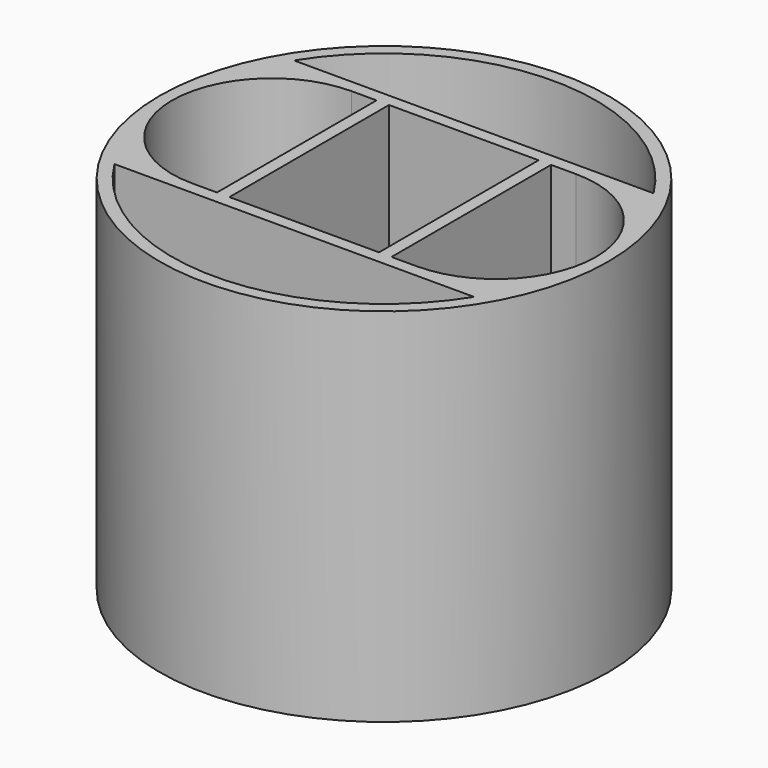
from build123d import *

# Parameters (mm, degrees)
F2_R     = 57.15
F3_DEPTH = 88.9
F0_R     = 57.15
F1_DEPTH = 3.175


# Not quite as in the source:
# - a feature names something its author has since deleted; it is built from what else it names


with BuildPart() as f3:
    # F2 (on Top) → F3 (new body)
    with BuildSketch(Plane.XY):
        with Locations((0, 25.4)):
            Circle(F2_R)
        with BuildLine():
            ThreePointArc((45.7905011984, -3.175), (0, -28.575), (-45.7905011984, -3.175))
            Line((-45.7905011984, -3.175), (45.7905011984, -3.175))
        make_face(mode=Mode.SUBTRACT)
        with BuildLine():
            Line((-22.225, 50.8), (-22.225, 0))
            Line((-22.225, 0), (-28.575, 0))
            ThreePointArc((-28.575, 0), (-53.975, 25.4), (-28.575, 50.8))
            Line((-28.575, 50.8), (-22.225, 50.8))
        make_face(mode=Mode.SUBTRACT)
        Polygon((19.05, 0), (0, 0), (-19.05, 0), (-19.05, 50.8), (0, 50.8), (19.05, 50.8), align=None, mode=Mode.SUBTRACT)
        with BuildLine():
            Line((28.575, 0), (22.225, 0))
            Line((22.225, 0), (22.225, 50.8))
            Line((22.225, 50.8), (28.575, 50.8))
            ThreePointArc((28.575, 50.8), (53.975, 25.4), (28.575, 0))
        make_face(mode=Mode.SUBTRACT)
        with BuildLine():
            Line((45.7905011984, 53.975), (-45.7905011984, 53.975))
            ThreePointArc((-45.7905011984, 53.975), (0, 79.375), (45.7905011984, 53.975))
        make_face(mode=Mode.SUBTRACT)
    extrude(amount=F3_DEPTH)

    # F0 (on face) → F1 (join)
    with BuildSketch(Plane(origin=(0, 0, 0), x_dir=(1, 0, 0), z_dir=(0, 0, -1))):
        with Locations((0, -25.4)):
            Circle(F0_R)
    extrude(amount=F1_DEPTH)


solid = f3.part
